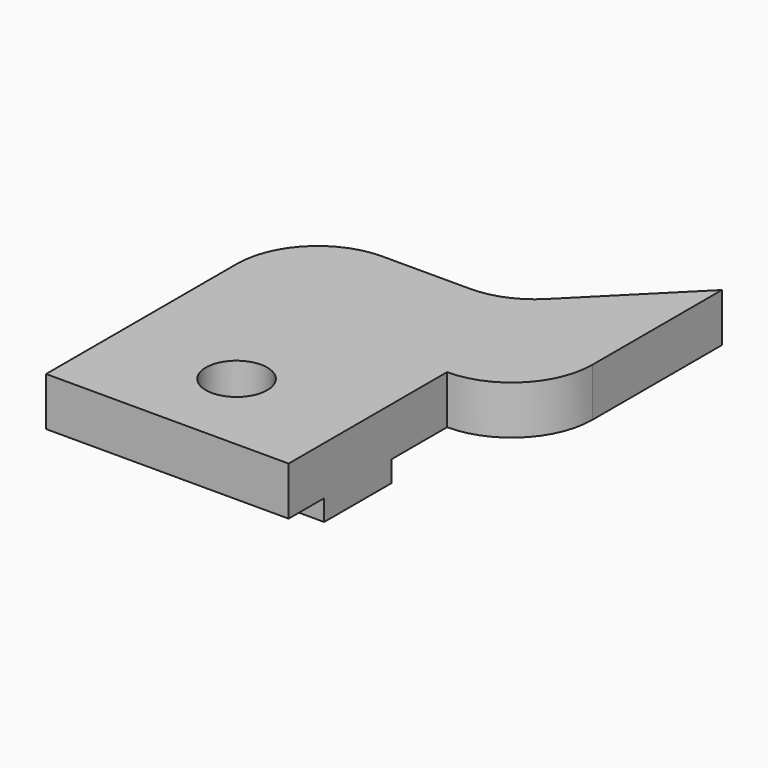
from build123d import *

# Parameters (mm, degrees)
F0_W     = 15
F0_H     = 2.75
F0_H_2   = 5.2
F0_R     = 1.9
F0_H_3   = 4.3
F1_DEPTH = 3
F2_DEPTH = 1.3
F3_R     = 4.99999


# Not quite as in the source:
# - a fillet or chamfer is up to 0.001 mm smaller than in the source, because OpenCascade refuses the exact size
# - a feature names something its author has since deleted; it is built from what else it names


with BuildPart() as f1:
    # F0 (on Top) → F1 (new body)
    with BuildSketch(Plane.XY):
        with Locations((0, 8.825)):
            Rectangle(F0_W, F0_H)
        with Locations((0, 12.8)):
            Rectangle(F0_W, F0_H_2)
        with Locations((0, 12.8)):
            Circle(F0_R, mode=Mode.SUBTRACT)
        with Locations((0, 17.55)):
            Rectangle(F0_W, F0_H_3)
        Polygon((-7.5, 27.2), (-7.5, 19.7), (7.5, 19.7), (12.5, 19.7), (12.5, 34.7), (5, 27.2), align=None)
    extrude(amount=F1_DEPTH)

    # F0 (on Top) → F2 (join)
    with BuildSketch(Plane.XY):
        with Locations((0, 12.8)):
            Rectangle(F0_W, F0_H_2)
        with Locations((0, 12.8)):
            Circle(F0_R, mode=Mode.SUBTRACT)
    extrude(amount=-F2_DEPTH)

    # F3 (radius 5 in the source; OpenCascade refuses exactly that, so slightly less here)
    f3_edges = [f1.edges().sort_by_distance(p)[0] for p in [
        (12.5, 19.7, 1.5),
        (-7.5, 27.2, 1.5),
        (5, 27.2, 1.5),
    ]]
    fillet(f3_edges, radius=F3_R)


solid = f1.part
